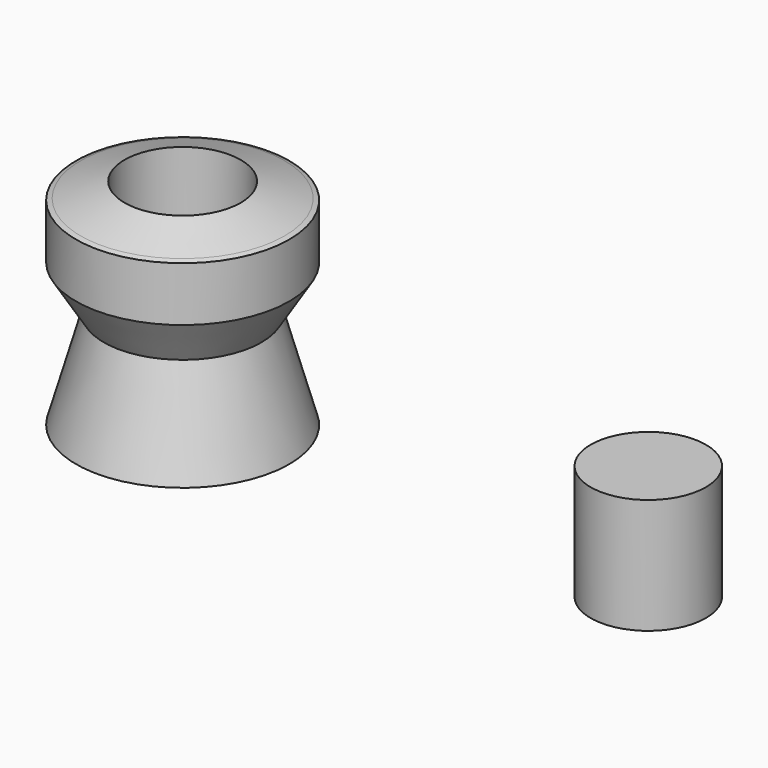
from build123d import *

# Parameters (mm, degrees)
F0_W = 5
F0_H = 10


# Not quite as in the source:
# - a feature names something its author has since deleted; it is built from what else it names


with BuildPart() as f1:
    # F0 (on Front) → F1 (revolve)
    with BuildSketch(Plane.XZ):
        Polygon((0, 10.3233849324), (0, 0), (9.254683698, 0), (6.8422881923, 8.5244880731), (9.254683698, 12.4379033223), (9.254683698, 14.0870045941), (9.254683698, 17.1659647299), (8.8474118947, 17.3053085763), (5.0441742836, 18.6065470946), (5.0441742836, 11.2733849324), (5.0441742836, 10.3233849324), align=None)
    revolve(axis=Axis((0, 0, 10.1661796476), (0, 0, 1)))


with BuildPart() as f2:
    # F0 (on Front) → F2 (revolve)
    with BuildSketch(Plane.XZ):
        with Locations((42.9124666942, 5)):
            Rectangle(F0_W, F0_H)
    revolve(axis=Axis((40.4124666942, 0, 5), (0, 0, -1)))


solid = Compound([f1.part, f2.part])
